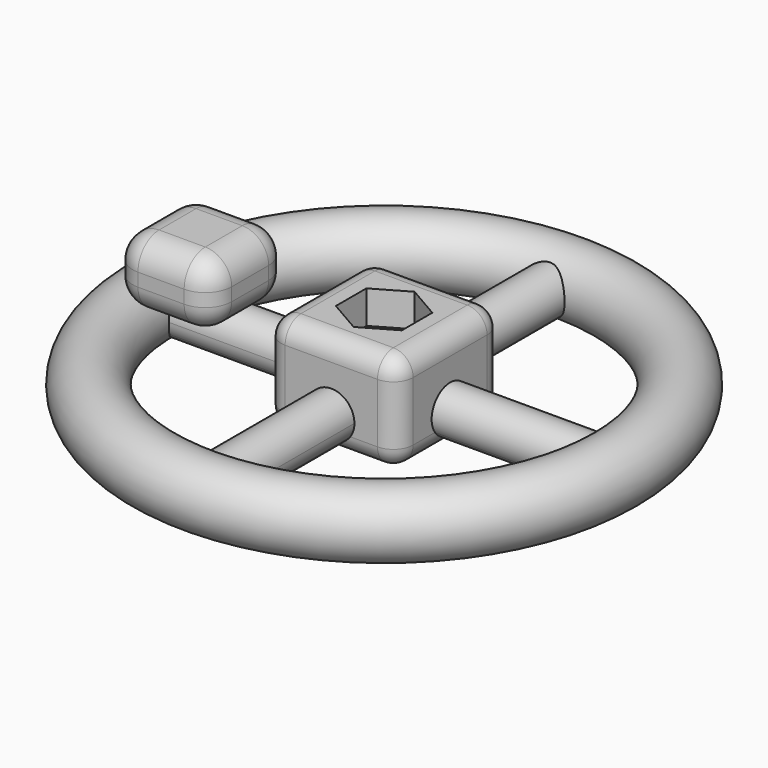
from build123d import *

# Parameters (mm, degrees)
F0_R           = 5
F3_W           = 20
F3_H           = 20
F4_DEPTH       = 10
F4_DEPTH_BACK  = 5
F5_R           = 3
F7_DEPTH       = 5
F8_R           = 3.4
F9_DEPTH       = 10.0010001
F11_DEPTH      = 25
F13_DEPTH      = 25
F15_DEPTH      = 25
F17_DEPTH      = 25
F21_W          = 15
F21_H          = 15
F22_DEPTH      = 5
F22_DEPTH_BACK = 5
F23_R          = 4


# Not quite as in the source:
# - the program builds the solid bodies; features that only make, move or delete a surface that nothing else refers to are left out


with BuildPart() as f2:
    # F0 (on Front) → F2 (revolve)
    with BuildSketch(Plane.XZ):
        with Locations((35, 0)):
            Circle(F0_R)
    revolve(axis=Axis((0, 0, 0), (0, 0, 1)))


with BuildPart() as f4:
    # F3 (on Top) → F4 (new body, two sides)
    with BuildSketch(Plane.XY) as f4_sk:
        Rectangle(F3_W, F3_H)
    extrude(amount=F4_DEPTH)
    extrude(f4_sk.sketch, amount=-F4_DEPTH_BACK)

    # F5
    f5_edges = [f4.edges().sort_by_distance(p)[0] for p in [
        (-10, 0, 10),
        (0, -10, 10),
        (10, 0, 10),
        (0, 10, 10),
        (10, -10, 2.5),
        (-10, -10, 2.5),
        (10, 10, 2.5),
        (-10, 10, 2.5),
        (0, -10, -5),
        (10, 0, -5),
        (0, 10, -5),
        (-10, 0, -5),
    ]]
    fillet(f5_edges, radius=F5_R)

    # F6 (on face) → F7 (cut)
    with BuildSketch(Plane.XY.offset(10)):
        Polygon((0, -5.7735026919), (5, -2.8867513459), (5, 2.8867513459), (0, 5.7735026919), (-5, 2.8867513459), (-5, -2.8867513459), align=None)
    extrude(amount=-F7_DEPTH, mode=Mode.SUBTRACT)

    # F8 (on face) → F9 (cut, through all)
    with BuildSketch(Plane.XY.offset(5)):
        Circle(F8_R)
    extrude(amount=-F9_DEPTH, mode=Mode.SUBTRACT)


with BuildPart() as f11:
    # F10 (on face) → F11 (new body)
    with BuildSketch(Plane.YZ.offset(10)):
        with BuildLine():
            Line((2.8722813233, -2), (-2.8722813233, -2))
            ThreePointArc((-2.8722813233, -2), (0, -3.5), (2.8722813233, -2))
        make_face()
        with BuildLine():
            ThreePointArc((2.8722813233, -2), (3.3393850206, -1.0480971731), (3.5, 0))
            ThreePointArc((3.5, 0), (-1.0480971731, 3.3393850206), (-2.8722813233, -2))
            Line((-2.8722813233, -2), (2.8722813233, -2))
        make_face()
    extrude(amount=F11_DEPTH)


with BuildPart() as f13:
    # F12 (on face) → F13 (new body)
    with BuildSketch(Plane(origin=(-10, 0, 0), x_dir=(0, -1, 0), z_dir=(-1, 0, 0))):
        with BuildLine():
            Line((2.8722813233, -2), (-2.8722813233, -2))
            ThreePointArc((-2.8722813233, -2), (0, -3.5), (2.8722813233, -2))
        make_face()
        with BuildLine():
            ThreePointArc((2.8722813233, -2), (3.3393850206, -1.0480971731), (3.5, 0))
            ThreePointArc((3.5, 0), (-1.0480971731, 3.3393850206), (-2.8722813233, -2))
            Line((-2.8722813233, -2), (2.8722813233, -2))
        make_face()
    extrude(amount=F13_DEPTH)


with BuildPart() as f15:
    # F14 (on face) → F15 (new body)
    with BuildSketch(Plane(origin=(0, 10, 0), x_dir=(-1, 0, 0), z_dir=(0, 1, 0))):
        with BuildLine():
            Line((2.8722813233, -2), (-2.8722813233, -2))
            ThreePointArc((-2.8722813233, -2), (0, -3.5), (2.8722813233, -2))
        make_face()
        with BuildLine():
            ThreePointArc((2.8722813233, -2), (3.3393850206, -1.0480971731), (3.5, 0))
            ThreePointArc((3.5, 0), (-1.0480971731, 3.3393850206), (-2.8722813233, -2))
            Line((-2.8722813233, -2), (2.8722813233, -2))
        make_face()
    extrude(amount=F15_DEPTH)


with BuildPart() as f17:
    # F16 (on face) → F17 (new body)
    with BuildSketch(Plane.XZ.offset(10)):
        with BuildLine():
            Line((2.8722813233, -2), (-2.8722813233, -2))
            ThreePointArc((-2.8722813233, -2), (0, -3.5), (2.8722813233, -2))
        make_face()
        with BuildLine():
            ThreePointArc((2.8722813233, -2), (3.3393850206, -1.0480971731), (3.5, 0))
            ThreePointArc((3.5, 0), (-1.0480971731, 3.3393850206), (-2.8722813233, -2))
            Line((-2.8722813233, -2), (2.8722813233, -2))
        make_face()
    extrude(amount=F17_DEPTH)


with BuildPart() as f22:
    # F21 (on offset) → F22 (new body, two sides)
    with BuildSketch(Plane.XY.offset(30)) as f22_sk:
        with Locations((0, -34.750711027)):
            Rectangle(F21_W, F21_H)
    extrude(amount=F22_DEPTH)
    extrude(f22_sk.sketch, amount=-F22_DEPTH_BACK)

    # F23
    f23_edges = [f22.edges().sort_by_distance(p)[0] for p in [
        (-7.5, -34.750711, 35),
        (0, -42.250711, 35),
        (7.5, -34.750711, 35),
        (0, -27.250711, 35),
        (0, -42.250711, 25),
        (-7.5, -34.750711, 25),
        (7.5, -34.750711, 25),
        (0, -27.250711, 25),
        (-7.5, -42.250711, 30),
        (7.5, -42.250711, 30),
        (7.5, -27.250711, 30),
        (-7.5, -27.250711, 30),
    ]]
    fillet(f23_edges, radius=F23_R)


solid = Compound([f2.part, f4.part, f11.part, f13.part, f15.part, f17.part, f22.part])
